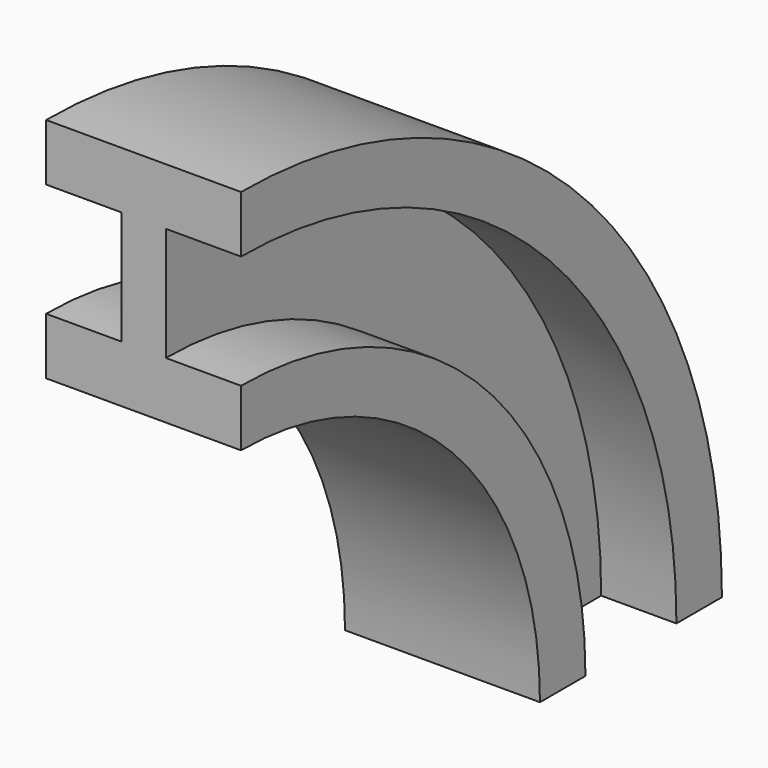
from build123d import *


# Not quite as in the source:
# - a feature of the source that left no trace in its solid (it failed there, or was rolled back) is left out


with BuildPart() as f2:
    # F2: sweep along a path in F1
    with BuildLine(Plane.YZ) as f2_path:
        ThreePointArc((0, 0), (269.4076836321, -111.5923163679), (381, -381))
    # F0 (on Front) → F2 (sweep)
    with BuildSketch(Plane.XZ):
        Polygon((76.2, 88.9), (0, 88.9), (-76.2, 88.9), (-76.2, 44.45), (-17.3748321831, 44.45), (-17.3748321831, 0), (-17.3748321831, -44.45), (-76.2, -44.45), (-76.2, -88.9), (0, -88.9), (76.2, -88.9), (76.2, -44.45), (17.3748321831, -44.45), (17.3748321831, 0), (17.3748321831, 44.45), (76.2, 44.45), align=None)
    sweep(path=f2_path.line)


solid = f2.part
